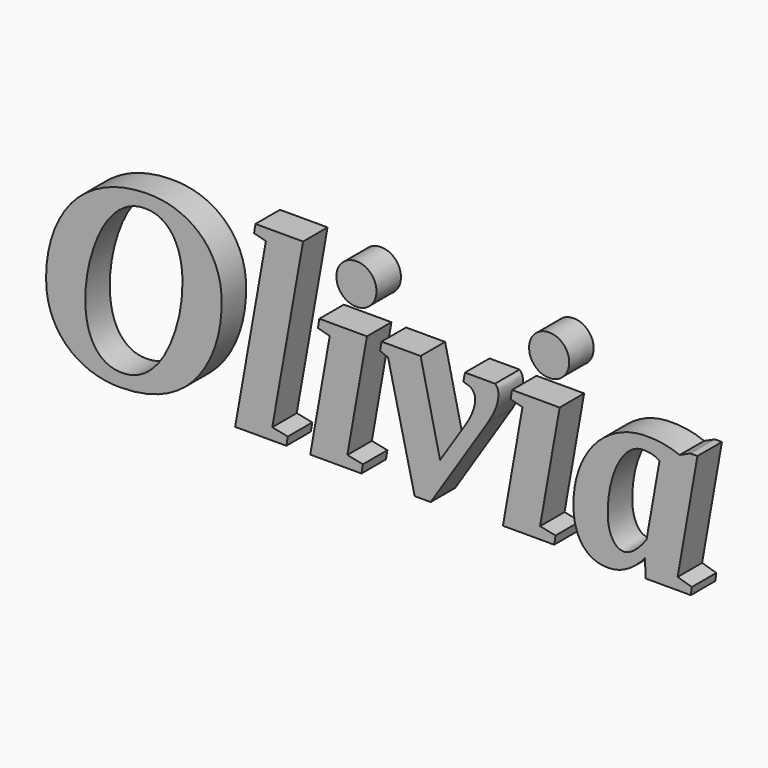
from build123d import *

# Parameters (mm, degrees)
F0_TEXT_SIZE = 87.1941757699
F1_DEPTH     = 10


# Not quite as in the source:
# - Text() gives the source's letters only with a copy of the font that has no kerning and outlines rounded to 1/6400 em; it was checked with that copy


with BuildPart() as f1:
    # F0 (on Front) → F1 (new body)
    with BuildSketch(Plane.XZ):
        with Locations((-110.2330945432, -33.7478313595)):
            Text('Olivia', F0_TEXT_SIZE, font='Tinos', font_style=FontStyle.BOLDITALIC, text_align=(TextAlign.LEFT, TextAlign.BOTTOM))
    extrude(amount=F1_DEPTH)


solid = f1.part
